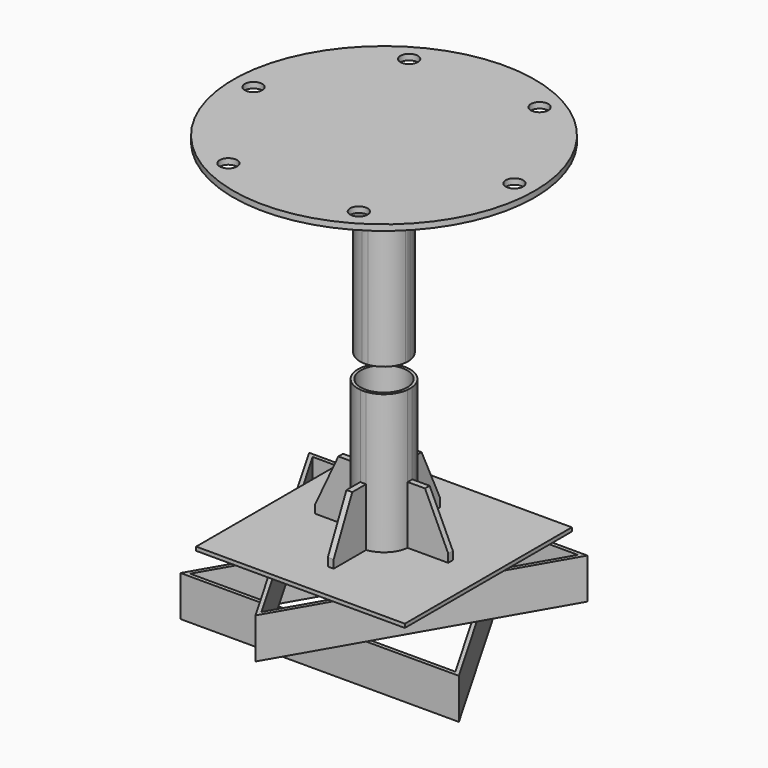
from build123d import *

# Parameters (mm, degrees)
F1_DEPTH    = 88.9
F4_DEPTH    = 88.9
F5_W        = 38.1
F5_H        = 330.2
F6_DEPTH    = 17.78
F7_W        = 457.2
F7_H        = 457.2
F8_DEPTH    = 8.255
F9_R        = 50.8
F10_DEPTH   = 304.8
F11_DEPTH   = 127
F12_SIZE2   = 108.9409515619
F12_SIZE    = 50.8
F12_2_SIZE2 = 108.9409515619
F12_2_SIZE  = 50.8
F12_3_SIZE2 = 108.9409515619
F12_3_SIZE  = 50.8
F12_4_SIZE2 = 108.9409515619
F12_4_SIZE  = 50.8
F15_DEPTH   = 127
F14_R       = 44.45
F16_DEPTH   = 406.4
F14_R_2     = 330.2
F17_DEPTH   = 12.7
F18_SIZE    = 88.9
F18_2_SIZE  = 88.9
F18_3_SIZE  = 88.9
F18_4_SIZE  = 88.9
F21_R       = 19.05
F22_DEPTH   = 960.756


with BuildPart() as f1:
    # F0 (on Top) → F1 (new body)
    with BuildSketch(Plane.XY):
        Polygon((-304.8, -175.976362049), (304.8, -175.976362049), (0, 351.952724098), align=None)
        Polygon((290.5019205835, -167.721362049), (-290.5019205835, -167.721362049), (0, 335.442724098), align=None, mode=Mode.SUBTRACT)
    extrude(amount=F1_DEPTH)


with BuildPart() as f4:
    # F3 (on offset) → F4 (new body)
    with BuildSketch(Plane.XY.offset(88.9)):
        Polygon((-304.8, 175.976362049), (0, -351.952724098), (304.8, 175.976362049), align=None)
        Polygon((0, -335.442724098), (-290.5019205835, 167.721362049), (290.5019205835, 167.721362049), align=None, mode=Mode.SUBTRACT)
    extrude(amount=F4_DEPTH)


with BuildPart() as f6:
    # F5 (on face) → F6 (new body)
    with BuildSketch(Plane.XY.offset(177.8)):
        with Locations((89.903781426, 2.621362049)):
            Rectangle(F5_W, F5_H)
    extrude(amount=F6_DEPTH)


with BuildPart() as f6b:
    # F5 (on face) → F6, piece 2 (new body)
    with BuildSketch(Plane.XY.offset(177.8)):
        with Locations((-80.8387121677, 2.621362049)):
            Rectangle(F5_W, F5_H)
    extrude(amount=F6_DEPTH)


with BuildPart() as f8:
    # F7 (on face) → F8 (new body)
    with BuildSketch(Plane.XY.offset(177.8)):
        Rectangle(F7_W, F7_H)
    extrude(amount=F8_DEPTH)


with BuildPart() as f10:
    # F9 (on face) → F10 (new body)
    with BuildSketch(Plane.XY.offset(186.055)):
        with BuildLine():
            Line((56.7961266285, -6.35), (56.7961266285, 6.35))
            ThreePointArc((56.7961266285, 6.35), (40.4111525448, 40.4111525448), (6.35, 56.7961266285))
            ThreePointArc((6.35, 56.7961266285), (0, 57.15), (-6.35, 56.7961266285))
            ThreePointArc((-6.35, 56.7961266285), (-40.4111525448, 40.4111525448), (-56.7961266285, 6.35))
            ThreePointArc((-56.7961266285, 6.35), (-57.15, 0), (-56.7961266285, -6.35))
            ThreePointArc((-56.7961266285, -6.35), (-40.4111525448, -40.4111525448), (-6.35, -56.7961266285))
            ThreePointArc((-6.35, -56.7961266285), (0, -57.15), (6.35, -56.7961266285))
            ThreePointArc((6.35, -56.7961266285), (40.4111525448, -40.4111525448), (56.7961266285, -6.35))
        make_face()
        Circle(F9_R, mode=Mode.SUBTRACT)
    extrude(amount=F10_DEPTH)


with BuildPart() as f11:
    # F9 (on face) → F11 (new body)
    with BuildSketch(Plane.XY.offset(186.055)):
        with BuildLine():
            ThreePointArc((-56.7961266285, -6.35), (-57.15, 0), (-56.7961266285, 6.35))
            Line((-56.7961266285, 6.35), (-145.6961266285, 6.35))
            Line((-145.6961266285, 6.35), (-145.6961266285, -6.35))
            Line((-145.6961266285, -6.35), (-56.7961266285, -6.35))
        make_face()
    extrude(amount=F11_DEPTH)

    # F12#3
    f12_3_edges = [f11.edges().sort_by_distance(p)[0] for p in [
        (-145.696127, 0, 313.055),
    ]]
    f12_3_side = f11.faces().sort_by_distance((-101.364095, 0, 313.055))[0]
    chamfer(f12_3_edges, length=F12_3_SIZE, length2=F12_3_SIZE2, reference=f12_3_side)


with BuildPart() as f11b:
    # F9 (on face) → F11, piece 2 (new body)
    with BuildSketch(Plane.XY.offset(186.055)):
        with BuildLine():
            Line((6.35, -145.6961266285), (6.35, -56.7961266285))
            ThreePointArc((6.35, -56.7961266285), (0, -57.15), (-6.35, -56.7961266285))
            Line((-6.35, -56.7961266285), (-6.35, -145.6961266285))
            Line((-6.35, -145.6961266285), (6.35, -145.6961266285))
        make_face()
    extrude(amount=F11_DEPTH)

    # F12#2
    f12_2_edges = [f11b.edges().sort_by_distance(p)[0] for p in [
        (0, -145.696127, 313.055),
    ]]
    f12_2_side = f11b.faces().sort_by_distance((0, -101.364095, 313.055))[0]
    chamfer(f12_2_edges, length=F12_2_SIZE, length2=F12_2_SIZE2, reference=f12_2_side)


with BuildPart() as f11c:
    # F9 (on face) → F11, piece 3 (new body)
    with BuildSketch(Plane.XY.offset(186.055)):
        with BuildLine():
            ThreePointArc((-6.35, 56.7961266285), (0, 57.15), (6.35, 56.7961266285))
            Line((6.35, 56.7961266285), (6.35, 145.6961266285))
            Line((6.35, 145.6961266285), (-6.35, 145.6961266285))
            Line((-6.35, 145.6961266285), (-6.35, 56.7961266285))
        make_face()
    extrude(amount=F11_DEPTH)

    # F12#4
    f12_4_edges = [f11c.edges().sort_by_distance(p)[0] for p in [
        (0, 145.696127, 313.055),
    ]]
    f12_4_side = f11c.faces().sort_by_distance((0, 101.364095, 313.055))[0]
    chamfer(f12_4_edges, length=F12_4_SIZE, length2=F12_4_SIZE2, reference=f12_4_side)


with BuildPart() as f11d:
    # F9 (on face) → F11, piece 4 (new body)
    with BuildSketch(Plane.XY.offset(186.055)):
        with BuildLine():
            ThreePointArc((56.7961266285, 6.35), (57.0614630763, 3.1799263499), (57.15, 0))
            ThreePointArc((57.15, 0), (57.0614630763, -3.1799263499), (56.7961266285, -6.35))
            Line((56.7961266285, -6.35), (145.6961266285, -6.35))
            Line((145.6961266285, -6.35), (145.6961266285, 6.35))
            Line((145.6961266285, 6.35), (56.7961266285, 6.35))
        make_face()
    extrude(amount=F11_DEPTH)

    # F12
    f12_edges = [f11d.edges().sort_by_distance(p)[0] for p in [
        (145.696127, 0, 313.055),
    ]]
    f12_side = f11d.faces().sort_by_distance((101.364095, 0, 313.055))[0]
    chamfer(f12_edges, length=F12_SIZE, length2=F12_SIZE2, reference=f12_side)


with BuildPart() as f15:
    # F14 (on offset) → F15 (new body)
    with BuildSketch(Plane.XY.offset(948.055)):
        with BuildLine():
            ThreePointArc((-6.2950344052, 52.3277131818), (0.0553689291, 52.7049709162), (6.4049655948, 52.3143712638))
            Line((6.4049655948, 52.3143712638), (6.4049655948, 179.705))
            Line((6.4049655948, 179.705), (-6.2950344052, 179.705))
            Line((-6.2950344052, 179.705), (-6.2950344052, 52.3277131818))
        make_face()
    extrude(amount=-F15_DEPTH)

    # F18
    f18_edges = [f15.edges().sort_by_distance(p)[0] for p in [
        (0.054966, 179.705, 821.055),
    ]]
    chamfer(f18_edges, length=F18_SIZE)


with BuildPart() as f15b:
    # F14 (on offset) → F15, piece 2 (new body)
    with BuildSketch(Plane.XY.offset(948.055)):
        with BuildLine():
            ThreePointArc((-52.3277131818, -6.2950344052), (-52.7049709162, 0.0553689291), (-52.3143712638, 6.4049655948))
            Line((-52.3143712638, 6.4049655948), (-179.705, 6.4049655948))
            Line((-179.705, 6.4049655948), (-179.705, -6.2950344052))
            Line((-179.705, -6.2950344052), (-52.3277131818, -6.2950344052))
        make_face()
    extrude(amount=-F15_DEPTH)

    # F18#3
    f18_3_edges = [f15b.edges().sort_by_distance(p)[0] for p in [
        (-179.705, 0.054966, 821.055),
    ]]
    chamfer(f18_3_edges, length=F18_3_SIZE)


with BuildPart() as f15c:
    # F14 (on offset) → F15, piece 3 (new body)
    with BuildSketch(Plane.XY.offset(948.055)):
        with BuildLine():
            Line((6.2950344052, -179.705), (6.2950344052, -52.3277131818))
            ThreePointArc((6.2950344052, -52.3277131818), (-0.0553689291, -52.7049709162), (-6.4049655948, -52.3143712638))
            Line((-6.4049655948, -52.3143712638), (-6.4049655948, -179.705))
            Line((-6.4049655948, -179.705), (6.2950344052, -179.705))
        make_face()
    extrude(amount=-F15_DEPTH)

    # F18#4
    f18_4_edges = [f15c.edges().sort_by_distance(p)[0] for p in [
        (-0.054966, -179.705, 821.055),
    ]]
    chamfer(f18_4_edges, length=F18_4_SIZE)


with BuildPart() as f15d:
    # F14 (on offset) → F15, piece 4 (new body)
    with BuildSketch(Plane.XY.offset(948.055)):
        with BuildLine():
            ThreePointArc((52.3277131818, 6.2950344052), (52.6105937443, 3.1531652155), (52.705, 0))
            ThreePointArc((52.705, 0), (52.6072521733, -3.2084332267), (52.3143712638, -6.4049655948))
            Line((52.3143712638, -6.4049655948), (179.705, -6.4049655948))
            Line((179.705, -6.4049655948), (179.705, 6.2950344052))
            Line((179.705, 6.2950344052), (52.3277131818, 6.2950344052))
        make_face()
    extrude(amount=-F15_DEPTH)

    # F18#2
    f18_2_edges = [f15d.edges().sort_by_distance(p)[0] for p in [
        (179.705, -0.054966, 821.055),
    ]]
    chamfer(f18_2_edges, length=F18_2_SIZE)


with BuildPart() as f16:
    # F14 (on offset) → F16 (new body)
    with BuildSketch(Plane.XY.offset(948.055)):
        with BuildLine():
            ThreePointArc((52.3143712638, -6.4049655948), (52.6072521733, -3.2084332267), (52.705, 0))
            ThreePointArc((52.705, 0), (52.6105937443, 3.1531652155), (52.3277131818, 6.2950344052))
            ThreePointArc((52.3277131818, 6.2950344052), (37.3071940824, 37.2288905919), (6.4049655948, 52.3143712638))
            ThreePointArc((6.4049655948, 52.3143712638), (0.0553689291, 52.7049709162), (-6.2950344052, 52.3277131818))
            ThreePointArc((-6.2950344052, 52.3277131818), (-37.2288905919, 37.3071940824), (-52.3143712638, 6.4049655948))
            ThreePointArc((-52.3143712638, 6.4049655948), (-52.7049709162, 0.0553689291), (-52.3277131818, -6.2950344052))
            ThreePointArc((-52.3277131818, -6.2950344052), (-37.3071940824, -37.2288905919), (-6.4049655948, -52.3143712638))
            ThreePointArc((-6.4049655948, -52.3143712638), (-0.0553689291, -52.7049709162), (6.2950344052, -52.3277131818))
            ThreePointArc((6.2950344052, -52.3277131818), (37.2288905919, -37.3071940824), (52.3143712638, -6.4049655948))
        make_face()
        Circle(F14_R, mode=Mode.SUBTRACT)
    extrude(amount=-F16_DEPTH)


with BuildPart() as f17:
    # F14 (on offset) → F17 (new body)
    with BuildSketch(Plane.XY.offset(948.055)):
        Circle(F14_R_2)
        with BuildLine():
            ThreePointArc((6.4049655948, 52.3143712638), (37.3071940824, 37.2288905919), (52.3277131818, 6.2950344052))
            Line((52.3277131818, 6.2950344052), (179.705, 6.2950344052))
            Line((179.705, 6.2950344052), (179.705, -6.4049655948))
            Line((179.705, -6.4049655948), (52.3143712638, -6.4049655948))
            ThreePointArc((52.3143712638, -6.4049655948), (37.2288905919, -37.3071940824), (6.2950344052, -52.3277131818))
            Line((6.2950344052, -52.3277131818), (6.2950344052, -179.705))
            Line((6.2950344052, -179.705), (-6.4049655948, -179.705))
            Line((-6.4049655948, -179.705), (-6.4049655948, -52.3143712638))
            ThreePointArc((-6.4049655948, -52.3143712638), (-37.3071940824, -37.2288905919), (-52.3277131818, -6.2950344052))
            Line((-52.3277131818, -6.2950344052), (-179.705, -6.2950344052))
            Line((-179.705, -6.2950344052), (-179.705, 6.4049655948))
            Line((-179.705, 6.4049655948), (-52.3143712638, 6.4049655948))
            ThreePointArc((-52.3143712638, 6.4049655948), (-37.2288905919, 37.3071940824), (-6.2950344052, 52.3277131818))
            Line((-6.2950344052, 52.3277131818), (-6.2950344052, 179.705))
            Line((-6.2950344052, 179.705), (6.4049655948, 179.705))
            Line((6.4049655948, 179.705), (6.4049655948, 52.3143712638))
        make_face(mode=Mode.SUBTRACT)
        with BuildLine():
            ThreePointArc((52.3143712638, -6.4049655948), (52.6072521733, -3.2084332267), (52.705, 0))
            ThreePointArc((52.705, 0), (52.6105937443, 3.1531652155), (52.3277131818, 6.2950344052))
            ThreePointArc((52.3277131818, 6.2950344052), (37.3071940824, 37.2288905919), (6.4049655948, 52.3143712638))
            ThreePointArc((6.4049655948, 52.3143712638), (0.0553689291, 52.7049709162), (-6.2950344052, 52.3277131818))
            ThreePointArc((-6.2950344052, 52.3277131818), (-37.2288905919, 37.3071940824), (-52.3143712638, 6.4049655948))
            ThreePointArc((-52.3143712638, 6.4049655948), (-52.7049709162, 0.0553689291), (-52.3277131818, -6.2950344052))
            ThreePointArc((-52.3277131818, -6.2950344052), (-37.3071940824, -37.2288905919), (-6.4049655948, -52.3143712638))
            ThreePointArc((-6.4049655948, -52.3143712638), (-0.0553689291, -52.7049709162), (6.2950344052, -52.3277131818))
            ThreePointArc((6.2950344052, -52.3277131818), (37.2288905919, -37.3071940824), (52.3143712638, -6.4049655948))
        make_face()
        Circle(F14_R, mode=Mode.SUBTRACT)
        with BuildLine():
            Line((6.2950344052, -179.705), (6.2950344052, -52.3277131818))
            ThreePointArc((6.2950344052, -52.3277131818), (-0.0553689291, -52.7049709162), (-6.4049655948, -52.3143712638))
            Line((-6.4049655948, -52.3143712638), (-6.4049655948, -179.705))
            Line((-6.4049655948, -179.705), (6.2950344052, -179.705))
        make_face()
        with BuildLine():
            ThreePointArc((52.3277131818, 6.2950344052), (52.6105937443, 3.1531652155), (52.705, 0))
            ThreePointArc((52.705, 0), (52.6072521733, -3.2084332267), (52.3143712638, -6.4049655948))
            Line((52.3143712638, -6.4049655948), (179.705, -6.4049655948))
            Line((179.705, -6.4049655948), (179.705, 6.2950344052))
            Line((179.705, 6.2950344052), (52.3277131818, 6.2950344052))
        make_face()
        with BuildLine():
            ThreePointArc((-52.3277131818, -6.2950344052), (-52.7049709162, 0.0553689291), (-52.3143712638, 6.4049655948))
            Line((-52.3143712638, 6.4049655948), (-179.705, 6.4049655948))
            Line((-179.705, 6.4049655948), (-179.705, -6.2950344052))
            Line((-179.705, -6.2950344052), (-52.3277131818, -6.2950344052))
        make_face()
        with BuildLine():
            ThreePointArc((-6.2950344052, 52.3277131818), (0.0553689291, 52.7049709162), (6.4049655948, 52.3143712638))
            Line((6.4049655948, 52.3143712638), (6.4049655948, 179.705))
            Line((6.4049655948, 179.705), (-6.2950344052, 179.705))
            Line((-6.2950344052, 179.705), (-6.2950344052, 52.3277131818))
        make_face()
        Circle(F14_R)
    extrude(amount=F17_DEPTH)

    # F21 (on face) → F22 (cut, through all)
    with BuildSketch(Plane.XY.offset(960.755)):
        with Locations((-285.75, 0)):
            Circle(F21_R)
        with Locations((-142.875, 247.4667591314)):
            Circle(F21_R)
        with Locations((142.875, 247.4667591314)):
            Circle(F21_R)
        with Locations((285.75, 0)):
            Circle(F21_R)
        with Locations((142.875, -247.4667591314)):
            Circle(F21_R)
        with Locations((-142.875, -247.4667591314)):
            Circle(F21_R)
    extrude(amount=-F22_DEPTH, mode=Mode.SUBTRACT)


solid = Compound([f1.part, f4.part, f8.part, f10.part, f11.part, f11b.part, f11c.part, f11d.part, f15.part, f15b.part, f15c.part, f15d.part, f16.part, f17.part])
